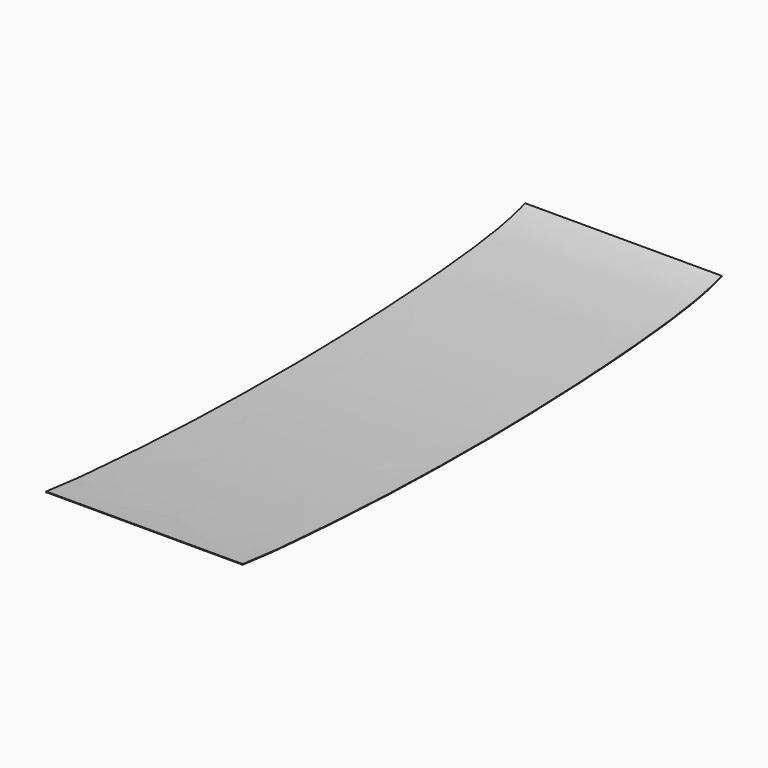
from build123d import *

# Parameters (mm, degrees)
F1_DEPTH = 1000


# Not quite as in the source:
# - the dataset's text gives a spline's control points without its knots; the knots are read off the source's solid


with BuildPart() as f1:
    # F0 (on Right) → F1 (new body)
    with BuildSketch(Plane.YZ):
        with BuildLine():
            Line((-1523.3073018893, 74.9343461632), (-1524, 72))
            add(Edge.make_bspline(
                [(-1524, 72), (-1523.5133752437, 71.8851246477), (-1408.7912269509, 59.1603797095), (-1328.1228770954, 51.1281516651), (-1222.9492078542, 42.3479525491), (-1124.2665744342, 37.4932045799), (-1023.94309645, 29.6764155139), (-924.0349531775, 23.805994689), (-823.9918225167, 19.1036206425), (-724.0143825979, 13.7803509145), (-624.0088625202, 9.7776519647), (-523.9984371896, 7.1107007848), (-424.0073790506, 3.7798389716), (-324.0036932597, 1.7707717723), (-223.9995081657, 1.1373887456), (-124.0016068592, -0.3202987771), (-23.9998974277, 0.1438353394), (76.0011965648, -0.2550497721), (176.0034437181, 0.8764133936), (276.0075220578, 2.7497464803), (375.9981147016, 6.1254124825), (476.0100095315, 8.748896998), (576.0101158316, 12.8806862016), (676.01688664, 17.7313952533), (775.9937905409, 24.1977156997), (876.0403182227, 29.4795593065), (976.0215348454, 37.8963611687), (1076.0108845518, 46.9469689387), (1176.1156760629, 56.3324859418), (1276.010139981, 69.7794335028), (1376.656372399, 84.6659141086), (1465.3163658887, 105.5732382543), (1523.5373474307, 124.8103882913), (1524, 125)],
                knots=[0, 0, 0, 0, 0.0326122587, 0.0652075875, 0.097773832, 0.1303174015, 0.1628715045, 0.195415074, 0.2279497224, 0.2604843708, 0.2930117147, 0.3255333739, 0.3580550332, 0.3905726301, 0.4230877889, 0.4556029477, 0.4881172936, 0.5206316396, 0.5531467984, 0.5856643953, 0.6181860545, 0.6507077138, 0.6832350577, 0.7157697061, 0.7483132755, 0.780856845, 0.8134230895, 0.846003078, 0.8785984068, 0.9112492637, 0.9439697331, 0.9769424993, 1, 1, 1, 1], degree=3))
            Line((1524, 125), (1522.8611233363, 127.7788590595))
            add(Edge.make_bspline(
                [(-1523.3073018888, 74.9343461725), (-1523.299966013, 74.9334494555), (-1523.2198083262, 74.9236681323), (-1523.0351200087, 74.9014757296), (-1522.6949712277, 74.8613702834), (-1522.281011374, 74.813156599), (-1521.6336009067, 74.7384018158), (-1520.6500623089, 74.6258641857), (-1519.2045189445, 74.4617964753), (-1517.5064355015, 74.2701394867), (-1515.5683567762, 74.0523015901), (-1512.680829434, 73.7288028034), (-1508.5334622756, 73.2659376191), (-1502.7946376568, 72.6279918709), (-1494.2583209074, 71.682132641), (-1482.1756974645, 70.3488200369), (-1466.2047587167, 68.5956437129), (-1452.3256836261, 67.0806516811), (-1441.2740386393, 65.880408023), (-1433.110295965, 64.9972258273), (-1425.1671741123, 64.1417787294), (-1417.5539457503, 63.3263016521), (-1410.2645680047, 62.550346295), (-1403.2674425262, 61.8106531305), (-1396.537552623, 61.1046865763), (-1387.8849679605, 60.2047266193), (-1377.6045448121, 59.1505684), (-1365.9130286935, 57.9773109209), (-1354.6549083103, 56.8742434495), (-1343.6186911004, 55.8198394852), (-1334.4298058641, 54.9637077803), (-1326.9788664776, 54.2816929058), (-1319.4219800533, 53.5975555479), (-1309.7497353302, 52.7359840788), (-1297.8474540558, 51.7014775596), (-1285.7037319278, 50.6746117593), (-1273.3759770786, 49.6640131639), (-1260.9207157003, 48.6782064212), (-1248.3948317049, 47.7257583557), (-1235.8547686388, 46.8151675408), (-1223.3585059103, 45.9551603228), (-1210.958467136, 45.1536129726), (-1198.6360512018, 44.3973720368), (-1182.2910618753, 43.4328778427), (-1161.9811113189, 42.2779329609), (-1141.733960569, 41.1063438127), (-1125.514377756, 40.1091337443), (-1109.2611940969, 39.0534264768), (-1088.8967781433, 37.6417694976), (-1064.4117108032, 35.8744683374), (-1039.9082234454, 34.1036747602), (-1015.4214251664, 32.4076032925), (-990.958447719, 30.8310333233), (-958.3559041302, 28.8609077144), (-917.6121754818, 26.6253211678), (-876.8270537221, 24.6041738352), (-844.188299385, 23.0081359533), (-811.54426929, 21.3890427801), (-770.7520458388, 19.2783937286), (-721.8187015492, 16.848406052), (-672.8806295114, 14.7386593589), (-623.9358370332, 12.9462115971), (-574.9808229355, 11.4733209265), (-526.005041876, 10.0876614049), (-477.0295609147, 8.5440536124), (-428.0730344258, 7.0598197918), (-379.1200369386, 5.8823730897), (-338.321993088, 5.170826056), (-305.6824661006, 4.7689805871), (-281.1977082019, 4.5277185043), (-256.7090728957, 4.3115855209), (-232.2162939694, 4.090917505), (-207.720091849, 3.8255327577), (-183.2304126015, 3.5332370927), (-158.7452897195, 3.2602517037), (-134.2650097936, 3.0431645046), (-109.789727149, 2.9312776117), (-85.3078661826, 2.9166511186), (-60.8211370084, 2.9506965411), (-36.3294557589, 2.9965217861), (-11.8319116788, 3.0049639707), (20.8245232819, 2.9629113558), (53.4728917987, 2.9232405587), (86.1112098449, 3.0295774046), (118.7514076717, 3.2573873147), (151.3937591024, 3.6350222195), (184.0390320755, 4.1158963002), (216.6820920486, 4.6583832374), (249.3215868938, 5.3193530019), (281.9548960454, 6.1457238508), (306.4319130454, 6.8510522932), (330.912698975, 7.6042301044), (355.3968946507, 8.3739629036), (379.8869681746, 9.1246335871), (412.5383858368, 10.0673562858), (445.1814763671, 10.9979485556), (477.8134164694, 12.0480507811), (510.4424680253, 13.219496519), (543.0722476693, 14.546141989), (575.7029912522, 15.9825228687), (608.3323919445, 17.476149314), (640.9554853129, 19.0819651007), (673.5701704718, 20.8514395746), (698.0289966565, 22.2760567825), (722.4923256935, 23.7613806024), (746.959737701, 25.2647132772), (771.4337349653, 26.7476087341), (795.9120908224, 28.1603042561), (820.3810299488, 29.5500781189), (844.8414236935, 30.9849244209), (869.2900729699, 32.5242275408), (893.7266679632, 34.2414118441), (918.1642800725, 36.1240069203), (942.6011356283, 38.1293353831), (967.0388018344, 40.2233411953), (991.4778005947, 42.3655125472), (1015.9147151689, 44.5405937528), (1040.3515045877, 46.746238925), (1064.7887107091, 48.9789966315), (1089.228663198, 51.2285077169), (1113.6602743849, 53.5224089098), (1138.0784076469, 55.920271631), (1158.4110852375, 58.048971006), (1174.6645543039, 59.857159664), (1190.9102081788, 61.7452795294), (1211.2108926353, 64.2454213124), (1235.570404771, 67.4303974807), (1255.8779464019, 70.2061975732), (1272.1338804738, 72.4811643118), (1288.3982257573, 74.7835615356), (1308.7247768932, 77.7323016393), (1333.0723979903, 81.485575974), (1353.2913924311, 84.8735386822), (1369.4051137127, 87.7890406266), (1385.4686390166, 90.8581906426), (1401.4699791607, 94.1779880698), (1417.461902047, 97.7770766137), (1429.4633970103, 100.6235368057), (1441.485185036, 103.6244809482), (1451.5307548628, 106.2601599676), (1459.590003099, 108.4533381993), (1465.6473631861, 110.1414458804), (1470.707424904, 111.585053419), (1474.7632266714, 112.7623756546), (1478.8258008787, 113.9552751797), (1483.891963184, 115.4664616), (1491.8465926311, 117.8813247966), (1499.3896545379, 120.2240497146), (1506.1509067278, 122.359109234), (1510.7385187374, 123.8227237097), (1514.7503113394, 125.1147858794), (1517.5364822246, 126.0202934524), (1519.3847183518, 126.6249470601), (1520.5687849618, 127.014259456), (1521.3771361125, 127.2815712044), (1521.9104782112, 127.4588524771), (1522.2520650523, 127.5728961012), (1522.5331982652, 127.6672909291), (1522.7149253271, 127.7288044967), (1522.8136870439, 127.762538229), (1522.8494466826, 127.7748332421), (1522.8611233501, 127.7788590193)],
                knots=[0.0013085711, 0.0013085711, 0.0013085711, 0.0013085711, 0.001359821, 0.0018575015, 0.0023551821, 0.0028528626, 0.0033505431, 0.0043459042, 0.0053412653, 0.0063366264, 0.0073319874, 0.0083273485, 0.0103180707, 0.0123087928, 0.014299515, 0.0182809593, 0.0222624036, 0.0262438479, 0.02823457, 0.0302252922, 0.0322160143, 0.0342067365, 0.0361974586, 0.0381881808, 0.0401789029, 0.0421696251, 0.0461510694, 0.0501325137, 0.054113958, 0.0580954023, 0.0620768466, 0.0640675687, 0.0660582909, 0.0700397352, 0.0740211795, 0.0780026238, 0.0819840681, 0.0859655124, 0.0899469567, 0.093928401, 0.0979098453, 0.1018912896, 0.1058727339, 0.1098541782, 0.1178170668, 0.1257799554, 0.1297613997, 0.133742844, 0.1417057326, 0.1496686212, 0.1576315098, 0.1655943984, 0.1735572871, 0.1815201757, 0.1974459529, 0.2133717301, 0.2213346187, 0.2292975073, 0.2452232845, 0.2611490617, 0.2770748389, 0.2930006161, 0.3089263933, 0.3248521705, 0.3407779477, 0.356703725, 0.3726295022, 0.3885552794, 0.396518168, 0.4044810566, 0.4124439452, 0.4204068338, 0.4283697224, 0.436332611, 0.4442954996, 0.4522583882, 0.4602212768, 0.4681841654, 0.476147054, 0.4841099426, 0.4920728312, 0.5000357198, 0.5159614971, 0.5239243857, 0.5318872743, 0.5478130515, 0.5557759401, 0.5637388287, 0.5796646059, 0.5876274945, 0.5955903831, 0.6035532717, 0.6115161603, 0.6194790489, 0.6274419375, 0.6433677147, 0.6513306033, 0.6592934919, 0.6752192691, 0.6831821577, 0.6911450464, 0.7070708236, 0.7150337122, 0.7229966008, 0.7309594894, 0.738922378, 0.7468852666, 0.7548481552, 0.7628110438, 0.7707739324, 0.778736821, 0.7866997096, 0.7946625982, 0.8026254868, 0.8105883754, 0.818551264, 0.8265141526, 0.8344770412, 0.8424399298, 0.8504028184, 0.858365707, 0.8663285957, 0.8742914843, 0.8782729286, 0.8822543729, 0.8902172615, 0.8981801501, 0.9061430387, 0.910124483, 0.9141059273, 0.9220688159, 0.9300317045, 0.9379945931, 0.9419760374, 0.9459574817, 0.9539203703, 0.9579018146, 0.9618832589, 0.9658647032, 0.9698461475, 0.9718368697, 0.9738275918, 0.975818314, 0.976813675, 0.9778090361, 0.9797997583, 0.9817904804, 0.9857719247, 0.9877626469, 0.989753369, 0.9917440912, 0.9937348133, 0.9947301744, 0.9957255355, 0.9967208966, 0.9972185771, 0.9977162576, 0.9982139382, 0.9987116187, 0.998960459, 0.9990969818, 0.9990969818, 0.9990969818, 0.9990969818], degree=3))
        make_face()
    extrude(amount=F1_DEPTH)


solid = f1.part
